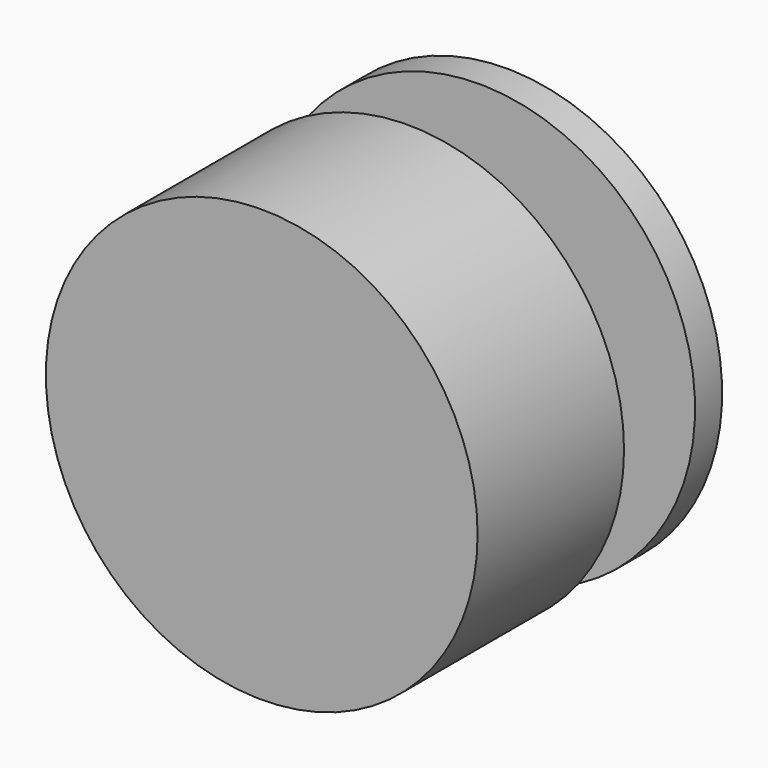
from build123d import *

# Parameters (mm, degrees)
F0_R     = 44
F1_DEPTH = 37.3
F5_START = 18.1
F4_R     = 44
F4_R_2   = 14
F5_DEPTH = 6.9


# Not quite as in the source:
# - the program builds the solid bodies; features that only make, move or delete a surface that nothing else refers to are left out


with BuildPart() as f1:
    # F0 (on Front) → F1 (new body)
    with BuildSketch(Plane.XZ):
        Circle(F0_R)
    extrude(amount=-F1_DEPTH)


with BuildPart() as f5:
    # F4 (on face) → F5 (new body)
    with BuildSketch(Plane(origin=(0, 37.3, 0), x_dir=(-1, 0, 0), z_dir=(0, 1, 0)).offset(F5_START)):
        Circle(F4_R)
        with Locations((1.7685926287, 0)):
            Circle(F4_R_2, mode=Mode.SUBTRACT)
    extrude(amount=F5_DEPTH)


solid = Compound([f1.part, f5.part])
